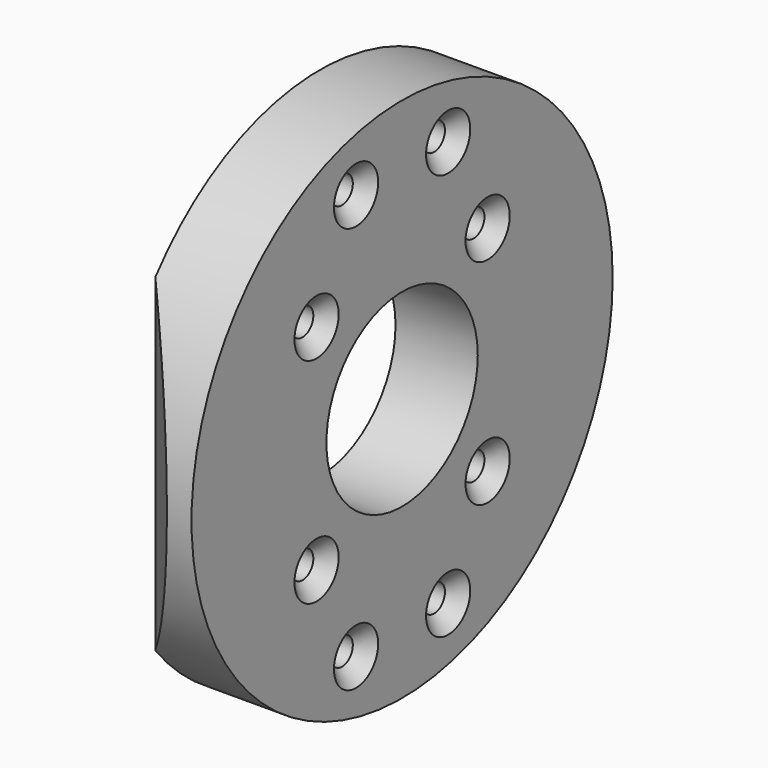
from build123d import *

# Parameters (mm, degrees)
F0_R           = 32
F1_DEPTH       = 10
F3_D           = 3.3
F3_CSINK_D     = 6.72
F3_CSINK_ANGLE = 90
F5_D           = 3.3
F5_CSINK_D     = 6.72
F5_CSINK_ANGLE = 90
F6_R           = 11.5
F7_DEPTH       = 10.001
F9_DEPTH       = 32.001
F9_DEPTH_BACK  = 32.001


with BuildPart() as f1:
    # F0 (on Right) → F1 (new body)
    with BuildSketch(Plane.YZ):
        Circle(F0_R)
    extrude(amount=F1_DEPTH)

    # F3 (through all)
    with Locations(Plane.YZ.offset(10)):
        with Locations((-13, 13), (13, 13), (13, -13), (-13, -13)):
            CounterSinkHole(F3_D / 2, F3_CSINK_D / 2, counter_sink_angle=F3_CSINK_ANGLE)

    # F5 (through all)
    with Locations(Plane.YZ.offset(10)):
        with Locations((-7, 24.7), (7, 24.7), (-7, -24.7), (7, -24.7)):
            CounterSinkHole(F5_D / 2, F5_CSINK_D / 2, counter_sink_angle=F5_CSINK_ANGLE)

    # F6 (on face) → F7 (cut, through all)
    with BuildSketch(Plane.YZ.offset(10)):
        Circle(F6_R)
    extrude(amount=-F7_DEPTH, mode=Mode.SUBTRACT)

    # F8 (on Top) → F9 (cut, two sides)
    with BuildSketch(Plane.XY) as f9_sk:
        Polygon((0, -25), (0, -32), (7, -32), align=None)
        Polygon((0, 32), (0, 25), (7, 32), align=None)
    extrude(amount=-F9_DEPTH, mode=Mode.SUBTRACT)
    extrude(f9_sk.sketch, amount=F9_DEPTH_BACK, mode=Mode.SUBTRACT)


solid = f1.part
